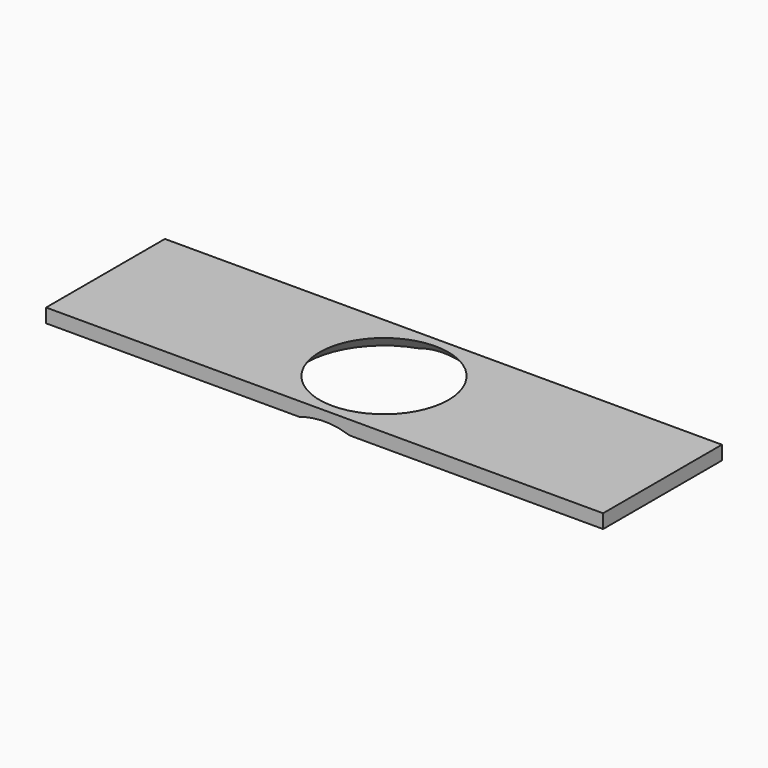
from build123d import *

# Parameters (mm, degrees)
F0_W     = 60
F0_H     = 16
F0_R     = 6.95
F1_DEPTH = 1.5


# Not quite as in the source:
# - a fillet or chamfer that OpenCascade refuses, or shapes differently, is made with other operations: its cross-section is extruded or revolved along the edge and cut away or added


with BuildPart() as f1:
    # F0 (on Top) → F1 (new body)
    with BuildSketch(Plane.XY):
        Rectangle(F0_W, F0_H)
        Circle(F0_R, mode=Mode.SUBTRACT)
    extrude(amount=F1_DEPTH)

    # F2: chamfer of 1.5 on 1 edges, made by hand

    # F2_s1 → F2_t2 (revolve, cut)
    with BuildSketch(Plane.XZ):
        Polygon((6.95, 1.5), (8.45, 0), (6.95, 0), align=None)
    revolve(axis=Axis((0, 0, 0), (0, 0, 1)), mode=Mode.SUBTRACT)


solid = f1.part
